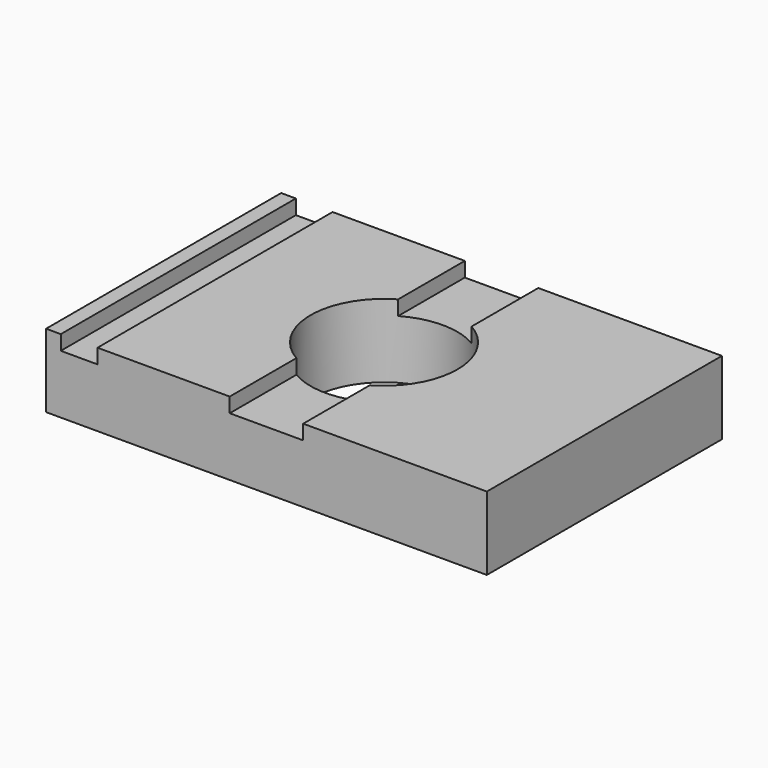
from build123d import *

# Parameters (mm, degrees)
F0_W     = 76.2
F0_H     = 50.8
F0_R     = 12.7
F1_DEPTH = 12.7
F2_W     = 6.35
F2_H     = 50.8
F3_DEPTH = 2.54


with BuildPart() as f1:
    # F0 (on Top) → F1 (new body)
    with BuildSketch(Plane.XY):
        Rectangle(F0_W, F0_H)
        Circle(F0_R, mode=Mode.SUBTRACT)
    extrude(amount=F1_DEPTH)

    # F2 (on face) → F3 (cut)
    with BuildSketch(Plane.XY.offset(12.7)):
        with Locations((-32.385, 0)):
            Rectangle(F2_W, F2_H)
        with BuildLine():
            Line((-6.35, -10.9985226281), (-6.35, -25.4))
            Line((-6.35, -25.4), (6.35, -25.4))
            Line((6.35, -25.4), (6.35, -10.9985226281))
            ThreePointArc((6.35, -10.9985226281), (0, -12.7), (-6.35, -10.9985226281))
        make_face()
        with BuildLine():
            Line((6.35, 25.4), (-6.35, 25.4))
            Line((-6.35, 25.4), (-6.35, 10.9985226281))
            ThreePointArc((-6.35, 10.9985226281), (0, 12.7), (6.35, 10.9985226281))
            Line((6.35, 10.9985226281), (6.35, 25.4))
        make_face()
    extrude(amount=-F3_DEPTH, mode=Mode.SUBTRACT)


solid = f1.part
